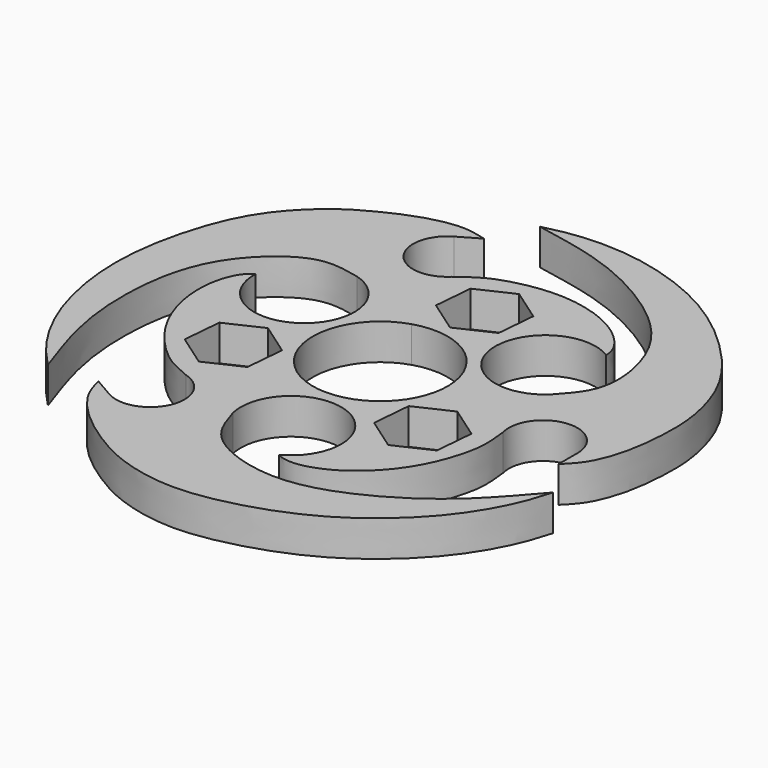
from build123d import *

# Parameters (mm, degrees)
F1_DEPTH = 5
F3_COUNT = 3
F5_DEPTH = 25


# Not quite as in the source:
# - a feature names something its author has since deleted; it is built from what else it names


with BuildPart() as f1:
    # F0 (on Top) → F1 (new body)
    with BuildSketch(Plane.XY):
        with BuildLine():
            ThreePointArc((19.3697792191, 5.4920897032), (7.5969915996, 9.8841483966), (18.2679687724, 16.5188265409))
            add(Edge.make_bspline(
                [(18.2679687724, 16.5188265409), (18.3496331671, 18.159304569), (15.0399422234, 22.4307572674), (5.8915424323, 25.1701629139), (-2.5645877448, 23.1556361007), (-4.2724416569, 21.9540160804), (-6.3755843906, 20.4204743588)],
                knots=[0, 0, 0, 0, 0.2303579847, 0.5244834011, 0.7878209886, 1, 1, 1, 1], degree=3))
            Line((-6.3755843906, 20.4204743588), (-2.8014574936, 8.9728387878))
            ThreePointArc((-2.8014574936, 8.9728387878), (6.3699775875, 6.9125527509), (9.1714350811, -2.0602860368))
            Line((9.1714350811, -2.0602860368), (20.8724397691, -4.6888186888))
            ThreePointArc((20.8724397691, -4.6888186888), (24.9046372172, 1.2367971287), (30.2800393035, -3.5041512456))
            Line((30.2800393035, -3.5041512456), (30.2800393035, -6.8021570911))
            add(Edge.make_bspline(
                [(-6.2640286051, 35.6329753995), (-4.879256488, 35.9717442203), (-1.585026432, 36.7719038353), (7.1656047644, 36.8306324291), (18.7097595399, 32.8325229218), (27.4190354107, 25.5475811449), (32.854692365, 18.5346088809), (34.9216993048, 10.9962495512), (34.9089688496, 5.8394018473), (34.4356780994, 0.7099122454), (32.81849257, -4.2517065064), (31.0670725646, -6.0125426883), (30.2800393035, -6.8021570911)],
                knots=[0, 0, 0, 0, 0.0814982335, 0.1926393238, 0.3258181235, 0.4537813969, 0.5666222077, 0.6709380758, 0.7568376371, 0.8431465468, 0.9290374106, 1, 1, 1, 1], degree=3))
            add(Edge.make_bspline(
                [(19.3697792191, 5.4920897032), (21.2657632456, 7.5222061316), (23.8510672601, 10.7996552166), (21.6544956387, 21.7849070989), (13.3248656234, 29.1499061822), (3.6795158583, 33.8104137468), (-3.1026823793, 35.0098141612), (-6.2640286051, 35.6329753995)],
                knots=[0, 0, 0, 0, 0.167152102, 0.3700687673, 0.5845137295, 0.7956301076, 1, 1, 1, 1], degree=3))
        make_face()
    extrude(amount=F1_DEPTH)

    # F3: F1 ×3 about axis
    f3_axis = Axis((0, 0, 27.9298778623), (0, 0, 1))


with BuildPart() as f1_1:
    add(f1.part)
    for i in range(1, F3_COUNT):
        add(f1.part.rotate(f3_axis, i * 360 / F3_COUNT))

    # F4 (on face) → F5 (cut)
    with BuildSketch(Plane.XY.offset(5)):
        Polygon((-3.5056654712, 14.0841332571), (0.9587131702, 10.958141679), (5.8980906096, 13.2614112055), (6.3730894075, 18.6906723101), (1.9087107662, 21.8166638882), (-3.0306666732, 19.5133943617), align=None)
        Polygon((13.0000523306, -14.8645934826), (17.9394297699, -12.5613239561), (18.4144285679, -7.1320628515), (13.9500499265, -4.0060712734), (9.0106724872, -6.3093407999), (8.5356736892, -11.7386019045), align=None)
        Polygon((-19.3731417381, -3.8260788275), (-19.8481405361, -9.2553399321), (-15.3837618947, -12.3813315102), (-10.4443844554, -10.0780619837), (-9.9693856574, -4.6488008791), (-14.4337642988, -1.522809301), align=None)
    extrude(amount=-F5_DEPTH, mode=Mode.SUBTRACT)


solid = f1_1.part
